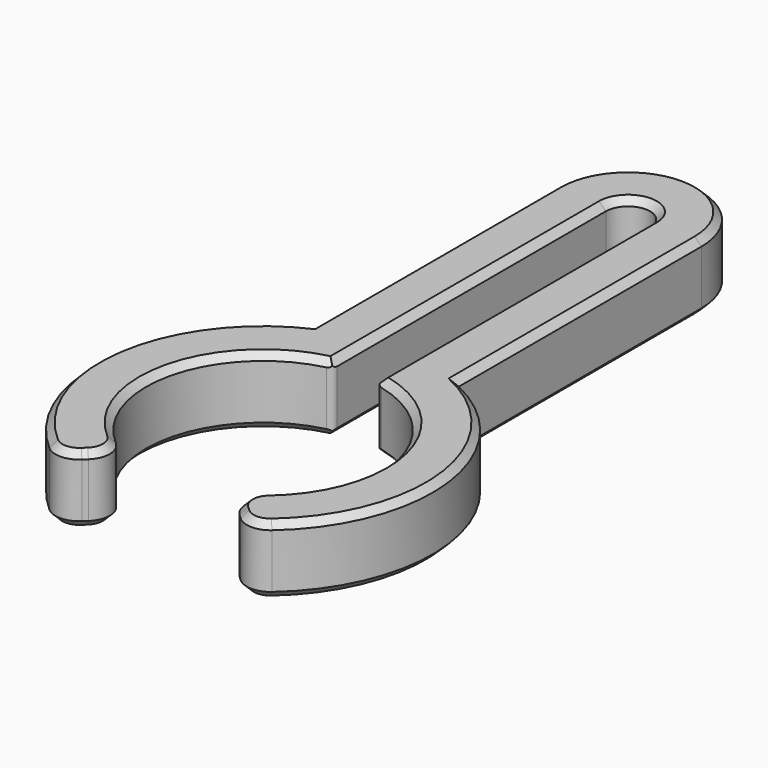
from build123d import *

# Parameters (mm, degrees)
F1_DEPTH = 10
F2_R     = 3.5
F3_SIZE  = 1
F4_R     = 1


# Not quite as in the source:
# - a feature names something its author has since deleted; it is built from what else it names


with BuildPart() as f1:
    # F0 (on Top) → F1 (new body)
    with BuildSketch(Plane.XY):
        with BuildLine():
            ThreePointArc((-44.3848475016, -14.7620242305), (-53.4374201274, 3.0310367894), (-39.6333784075, 17.4529133594))
            Line((-39.6333784075, 17.4529133594), (-39.6333784075, 67.7640176489))
            ThreePointArc((-39.6333784075, 67.7640176489), (-36.3720424684, 71.025353588), (-33.1107065292, 67.7640176489))
            Line((-33.1107065292, 67.7640176489), (-33.1107065292, 17.4529133594))
            ThreePointArc((-33.1107065292, 17.4529133594), (-19.3066648093, 3.0310367894), (-28.3592374351, -14.7620242305))
            Line((-28.3592374351, -14.7620242305), (-22.5229276093, -20.2994880054))
            ThreePointArc((-22.5229276093, -20.2994880054), (-11.4323530197, 2.249497469), (-25.5391483675, 23.0450718941))
            Line((-25.5391483675, 23.0450718941), (-25.5391483675, 67.7640176489))
            ThreePointArc((-25.5391483675, 67.7640176489), (-36.3720424684, 78.5969117497), (-47.2049365692, 67.7640176489))
            Line((-47.2049365692, 67.7640176489), (-47.2049365692, 23.0450718941))
            ThreePointArc((-47.2049365692, 23.0450718941), (-61.311731917, 2.249497469), (-50.2211573274, -20.2994880054))
            Line((-50.2211573274, -20.2994880054), (-44.3848475016, -14.7620242305))
        make_face()
    extrude(amount=F1_DEPTH)

    # F2
    f2_edges = [f1.edges().sort_by_distance(p)[0] for p in [
        (-50.221157, -20.299488, 5),
        (-44.384848, -14.762024, 5),
        (-28.359237, -14.762024, 5),
        (-22.522928, -20.299488, 5),
    ]]
    fillet(f2_edges, radius=F2_R)

    # F3
    f3_edges = [f1.edges().sort_by_distance(p)[0] for p in [
        (-53.038502, 4.962794, 10),
        (-61.149218, 3.844419, 10),
        (-47.204937, 45.404545, 10),
        (-39.633378, 42.608466, 10),
        (-36.372042, 78.596912, 10),
        (-36.372042, 71.025354, 10),
        (-33.110707, 42.608466, 10),
        (-25.539148, 45.404545, 10),
        (-19.705582, 4.962794, 10),
        (-11.594867, 3.844419, 0),
        (-25.539148, 45.404545, 0),
        (-39.633378, 42.608466, 0),
        (-53.038502, 4.962794, 0),
    ]]
    chamfer(f3_edges, length=F3_SIZE)

    # F4
    f4_edges = [f1.edges().sort_by_distance(p)[0] for p in [
        (-39.633378, 17.452913, 5),
        (-33.110707, 17.452913, 5),
    ]]
    fillet(f4_edges, radius=F4_R)


solid = f1.part
